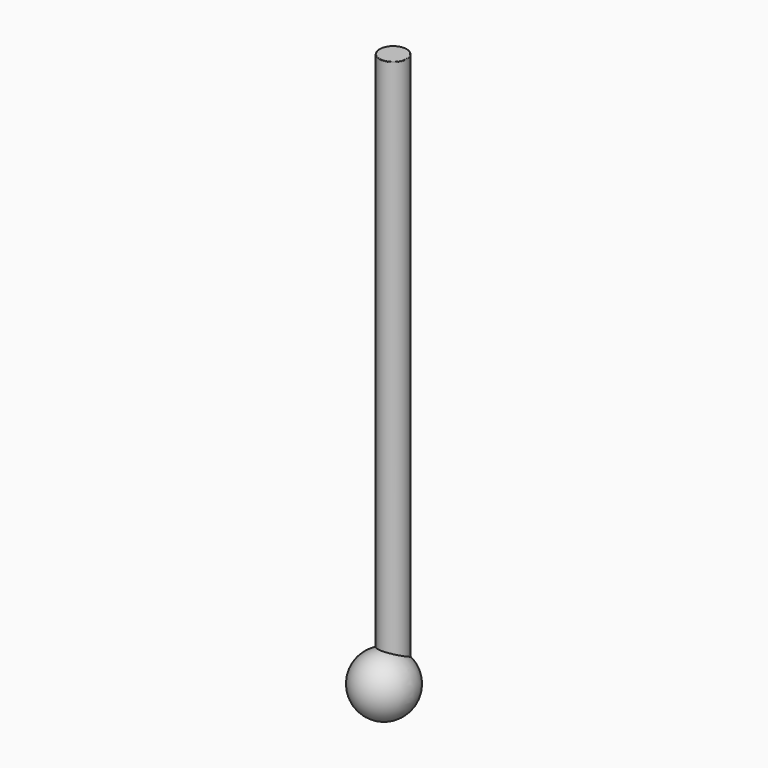
from build123d import *

# Parameters (mm, degrees)
F0_R     = 15.113
F1_DEPTH = 609.6
F2_R     = 0.635


# Not quite as in the source:
# - the program builds the solid bodies; features that only make, move or delete a surface that nothing else refers to are left out


with BuildPart() as f1:
    # F0 (on Top) → F1 (new body)
    with BuildSketch(Plane.XY):
        Circle(F0_R)
    extrude(amount=F1_DEPTH)

    # F2
    f2_edges = [f1.edges().sort_by_distance(p)[0] for p in [
        (-15.113, 0, 609.6),
    ]]
    fillet(f2_edges, radius=F2_R)


with BuildPart() as f7:
    # F6 (on offset) → F7 (revolve)
    with BuildSketch(Plane.XZ.offset(12.7)):
        with BuildLine():
            Line((0, 33.02), (0, -33.02))
            ThreePointArc((0, -33.02), (33.02, 0), (0, 33.02))
        make_face()
    revolve(axis=Axis((0, -12.7, 0), (0, 0, 1)))


solid = Compound([f1.part, f7.part])
